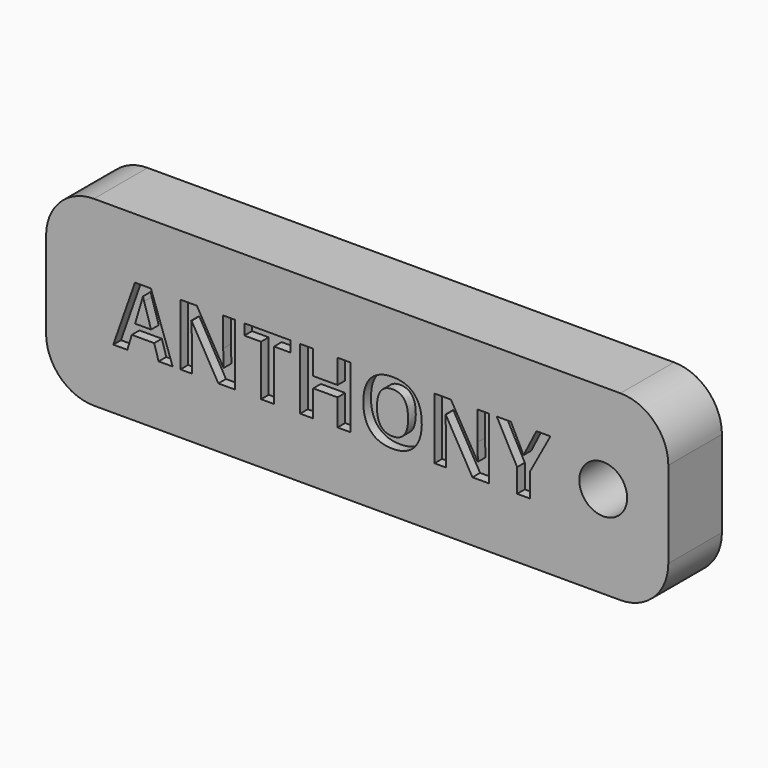
from build123d import *

# Parameters (mm, degrees)
F0_R         = 3.175
F1_DEPTH     = 8.89
F0_TEXT_SIZE = 11.4161838105
F2_DEPTH     = 7.62
F3_DEPTH     = 8.89


# Not quite as in the source:
# - Text() gives the source's letters only with a copy of the font that has no kerning and outlines rounded to 1/6400 em; it was checked with that copy


with BuildPart() as f1:
    # F0 (on Front) → F1 (new body)
    with BuildSketch(Plane.XZ):
        with BuildLine():
            Line((41.9675325871, 7.2492286563), (-27.8824674129, 7.2492286563))
            ThreePointArc((-27.8824674129, 7.2492286563), (-32.3725954735, 5.3893567168), (-34.2324674129, 0.8992286563))
            Line((-34.2324674129, 0.8992286563), (-34.2324674129, -10.564865002))
            ThreePointArc((-34.2324674129, -10.564865002), (-32.3725954735, -15.0549930626), (-27.8824674129, -16.914865002))
            Line((-27.8824674129, -16.914865002), (41.9675325871, -16.914865002))
            ThreePointArc((41.9675325871, -16.914865002), (46.4576606476, -15.0549930626), (48.3175325871, -10.564865002))
            Line((48.3175325871, -10.564865002), (48.3175325871, 0.8992286563))
            ThreePointArc((48.3175325871, 0.8992286563), (46.4576606476, 5.3893567168), (41.9675325871, 7.2492286563))
        make_face()
        Polygon((-17.4389670331, -8.9495686116), (-19.3012320172, -8.9495686116), (-19.8916627737, -7.0088173638), (-22.8634381218, -7.0088173638), (-23.4538688783, -8.9495686116), (-25.3161338624, -8.9495686116), (-22.4388987864, -0.7655918424), (-20.3269047814, -0.7655918424), align=None, mode=Mode.SUBTRACT)
        with BuildLine():
            Line((-9.1836391152, -0.7994836381), (-9.1836391152, -8.9495686116))
            Line((-9.1836391152, -8.9495686116), (-11.37947072, -8.9495686116))
            Line((-11.37947072, -8.9495686116), (-14.9256228161, -2.7848293539))
            Line((-14.9256228161, -2.7848293539), (-14.9755686203, -2.7848293539))
            add(Edge.make_bspline(
                [(-14.9755686203, -2.7848293539), (-14.8685418971, -4.4169868831), (-14.8685418971, -5.1144443627)],
                knots=[0, 0, 0, 1, 1, 1], degree=2))
            Line((-14.8685418971, -5.1144443627), (-14.8685418971, -8.9495686116))
            Line((-14.8685418971, -8.9495686116), (-16.4132942689, -8.9495686116))
            Line((-16.4132942689, -8.9495686116), (-16.4132942689, -0.7994836381))
            Line((-16.4132942689, -0.7994836381), (-14.2335166726, -0.7994836381))
            Line((-14.2335166726, -0.7994836381), (-10.6944996914, -6.9035744193))
            Line((-10.6944996914, -6.9035744193), (-10.6552565595, -6.9035744193))
            add(Edge.make_bspline(
                [(-10.6552565595, -6.9035744193), (-10.7390941594, -5.3142275794), (-10.7390941594, -4.6577970103)],
                knots=[0, 0, 0, 1, 1, 1], degree=2))
            Line((-10.7390941594, -4.6577970103), (-10.7390941594, -0.7994836381))
            Line((-10.7390941594, -0.7994836381), (-9.1836391152, -0.7994836381))
        make_face(mode=Mode.SUBTRACT)
        Polygon((-3.9874917027, -2.2372092868), (-3.9874917027, -8.9495686116), (-5.7159732828, -8.9495686116), (-5.7159732828, -2.2372092868), (-7.9296426748, -2.2372092868), (-7.9296426748, -0.7994836381), (-1.7756060894, -0.7994836381), (-1.7756060894, -2.2372092868), align=None, mode=Mode.SUBTRACT)
        Polygon((6.1568578801, -0.7994836381), (6.1568578801, -8.9495686116), (4.4337276362, -8.9495686116), (4.4337276362, -5.431956975), (1.2068719311, -5.431956975), (1.2068719311, -8.9495686116), (-0.521609649, -8.9495686116), (-0.521609649, -0.7994836381), (1.2068719311, -0.7994836381), (1.2068719311, -3.9942313263), (4.4337276362, -3.9942313263), (4.4337276362, -0.7994836381), align=None, mode=Mode.SUBTRACT)
        with BuildLine():
            add(Edge.make_bspline(
                [(14.6155365722, -1.7529133642), (15.6108850982, -2.8347751581), (15.6108850982, -4.8629315632)],
                knots=[0, 0, 0, 1, 1, 1], degree=2))
            add(Edge.make_bspline(
                [(15.6108850982, -4.8629315632), (15.6108850982, -6.8875204108), (14.607509568, -7.9747335409)],
                knots=[0, 0, 0, 1, 1, 1], degree=2))
            add(Edge.make_bspline(
                [(14.607509568, -7.9747335409), (13.6041340378, -9.061946671), (11.7311663813, -9.061946671)],
                knots=[0, 0, 0, 1, 1, 1], degree=2))
            add(Edge.make_bspline(
                [(11.7311663813, -9.061946671), (9.8581987249, -9.061946671), (8.8548231947, -7.9747335409)],
                knots=[0, 0, 0, 1, 1, 1], degree=2))
            add(Edge.make_bspline(
                [(8.8548231947, -7.9747335409), (7.8514476645, -6.8875204108), (7.8514476645, -4.8522288908)],
                knots=[0, 0, 0, 1, 1, 1], degree=2))
            add(Edge.make_bspline(
                [(7.8514476645, -4.8522288908), (7.8514476645, -2.8169373709), (8.8574988628, -1.7439944706)],
                knots=[0, 0, 0, 1, 1, 1], degree=2))
            add(Edge.make_bspline(
                [(8.8574988628, -1.7439944706), (9.8635500611, -0.6710515703), (11.7418690537, -0.6710515703)],
                knots=[0, 0, 0, 1, 1, 1], degree=2))
            add(Edge.make_bspline(
                [(11.7418690537, -0.6710515703), (13.6201880462, -0.6710515703), (14.6155365722, -1.7529133642)],
                knots=[0, 0, 0, 1, 1, 1], degree=2))
        make_face(mode=Mode.SUBTRACT)
        with BuildLine():
            Line((24.5297787001, -0.7994836381), (24.5297787001, -8.9495686116))
            Line((24.5297787001, -8.9495686116), (22.3339470953, -8.9495686116))
            Line((22.3339470953, -8.9495686116), (18.7877949992, -2.7848293539))
            Line((18.7877949992, -2.7848293539), (18.737849195, -2.7848293539))
            add(Edge.make_bspline(
                [(18.737849195, -2.7848293539), (18.8448759182, -4.4169868831), (18.8448759182, -5.1144443627)],
                knots=[0, 0, 0, 1, 1, 1], degree=2))
            Line((18.8448759182, -5.1144443627), (18.8448759182, -8.9495686116))
            Line((18.8448759182, -8.9495686116), (17.3001235464, -8.9495686116))
            Line((17.3001235464, -8.9495686116), (17.3001235464, -0.7994836381))
            Line((17.3001235464, -0.7994836381), (19.4799011427, -0.7994836381))
            Line((19.4799011427, -0.7994836381), (23.018918124, -6.9035744193))
            Line((23.018918124, -6.9035744193), (23.0581612558, -6.9035744193))
            add(Edge.make_bspline(
                [(23.0581612558, -6.9035744193), (22.9743236559, -5.3142275794), (22.9743236559, -4.6577970103)],
                knots=[0, 0, 0, 1, 1, 1], degree=2))
            Line((22.9743236559, -4.6577970103), (22.9743236559, -0.7994836381))
            Line((22.9743236559, -0.7994836381), (24.5297787001, -0.7994836381))
        make_face(mode=Mode.SUBTRACT)
        Polygon((27.4284191207, -0.7994836381), (29.117657569, -4.1547714112), (30.8175986895, -0.7994836381), (32.6798636736, -0.7994836381), (29.9756551335, -5.7780100467), (29.9756551335, -8.9495686116), (28.2596600044, -8.9495686116), (28.2596600044, -5.8333071871), (25.5554514643, -0.7994836381), align=None, mode=Mode.SUBTRACT)
        with Locations((39.6800078452, -4.687526729)):
            Circle(F0_R, mode=Mode.SUBTRACT)
    extrude(amount=F1_DEPTH)

    # F0 (on Front) → F2 (join)
    with BuildSketch(Plane.XZ):
        with Locations((-25.3161338624, -8.9495686116)):
            Text('ANTHONY', F0_TEXT_SIZE, font='Open Sans', font_style=FontStyle.BOLD, text_align=(TextAlign.LEFT, TextAlign.BOTTOM))
    extrude(amount=F2_DEPTH)

    # F0 (on Front) → F3 (join)
    with BuildSketch(Plane.XZ):
        with BuildLine():
            Line((-22.4281961141, -5.5603890428), (-20.3054994368, -5.5603890428))
            add(Edge.make_bspline(
                [(-20.3054994368, -5.5603890428), (-21.1242538695, -2.9239640941), (-21.2277130352, -2.5779110223)],
                knots=[0, 0, 0, 1, 1, 1], degree=2))
            add(Edge.make_bspline(
                [(-21.2277130352, -2.5779110223), (-21.331172201, -2.2318579506), (-21.375766669, -2.0320747339)],
                knots=[0, 0, 0, 1, 1, 1], degree=2))
            add(Edge.make_bspline(
                [(-21.375766669, -2.0320747339), (-21.5594958772, -2.7455862221), (-22.4281961141, -5.5603890428)],
                knots=[0, 0, 0, 1, 1, 1], degree=2))
        make_face()
        with BuildLine():
            add(Edge.make_bspline(
                [(10.1873058989, -2.8044509198), (9.6637668444, -3.4983408421), (9.6637668444, -4.8629315632)],
                knots=[0, 0, 0, 1, 1, 1], degree=2))
            add(Edge.make_bspline(
                [(9.6637668444, -4.8629315632), (9.6637668444, -6.229306063), (10.1819545627, -6.9205203171)],
                knots=[0, 0, 0, 1, 1, 1], degree=2))
            add(Edge.make_bspline(
                [(10.1819545627, -6.9205203171), (10.700142281, -7.6117345713), (11.7311663813, -7.6117345713)],
                knots=[0, 0, 0, 1, 1, 1], degree=2))
            add(Edge.make_bspline(
                [(11.7311663813, -7.6117345713), (13.7985659183, -7.6117345713), (13.7985659183, -4.8629315632)],
                knots=[0, 0, 0, 1, 1, 1], degree=2))
            add(Edge.make_bspline(
                [(13.7985659183, -4.8629315632), (13.7985659183, -2.1105609976), (11.7418690537, -2.1105609976)],
                knots=[0, 0, 0, 1, 1, 1], degree=2))
            add(Edge.make_bspline(
                [(11.7418690537, -2.1105609976), (10.7108449533, -2.1105609976), (10.1873058989, -2.8044509198)],
                knots=[0, 0, 0, 1, 1, 1], degree=2))
        make_face()
    extrude(amount=F3_DEPTH)


solid = f1.part
